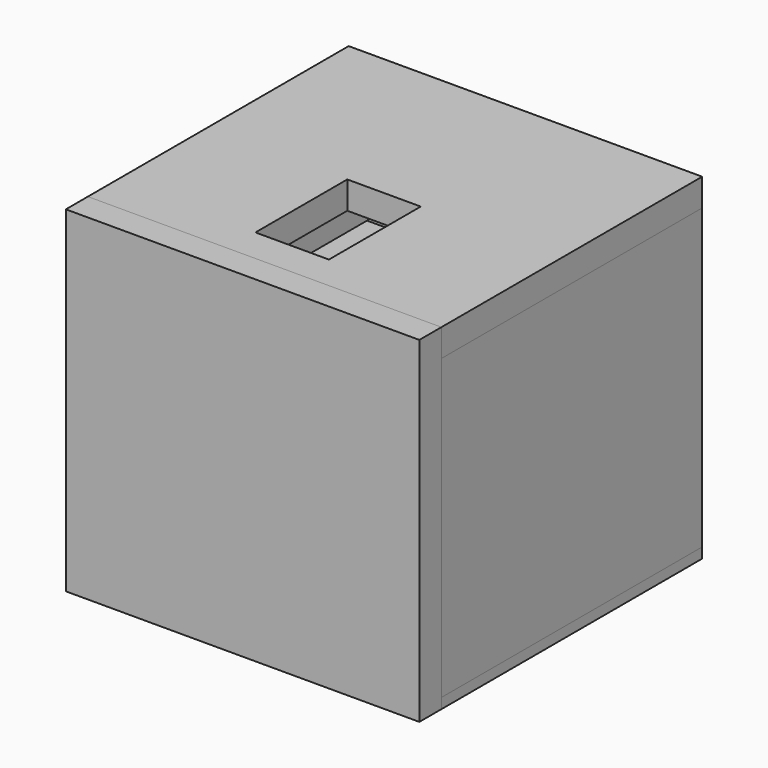
from build123d import *

# Parameters (mm, degrees)
F0_W      = 154
F0_H      = 146.5
F1_DEPTH  = 12
F2_W      = 142
F2_H      = 130
F3_DEPTH  = 12
F5_W      = 154
F5_H      = 142
F5_W_2    = 32
F5_H_2    = 50
F6_DEPTH  = 12
F7_W      = 154
F7_H      = 142
F8_DEPTH  = 4.5
F9_W      = 130
F9_H      = 130
F10_DEPTH = 4.5
F11_W     = 3
F11_H     = 3
F12_DEPTH = 142
F14_W     = 136
F14_H     = 137
F15_DEPTH = 3


# Not quite as in the source:
# - a feature names something its author has since deleted; it is built from what else it names


with BuildPart() as f1:
    # F0 (on Front) → F1 (new body)
    with BuildSketch(Plane.XZ):
        with Locations((0, 3.75)):
            Rectangle(F0_W, F0_H)
    extrude(amount=F1_DEPTH)


with BuildPart() as f3:
    # F2 (on face) → F3 (new body)
    with BuildSketch(Plane.YZ.offset(77)):
        with Locations((71, 0)):
            Rectangle(F2_W, F2_H)
    extrude(amount=-F3_DEPTH)

    # F11 (on face) → F12 (cut)
    with BuildSketch(Plane(origin=(0, 142, 0), x_dir=(-1, 0, 0), z_dir=(0, 1, 0))):
        with Locations((-66.5, 14.5)):
            Rectangle(F11_W, F11_H)
        with Locations((-66.5, -28.5)):
            Rectangle(F11_W, F11_H)
    extrude(amount=-F12_DEPTH, mode=Mode.SUBTRACT)


with BuildPart() as f4_1:
    # F4: instance of F1
    add(f1.part.mirror(Plane.YZ))


with BuildPart() as f6:
    # F5 (on face) → F6 (new body)
    with BuildSketch(Plane.XY.offset(77)):
        with Locations((0, 71)):
            Rectangle(F5_W, F5_H)
        with Locations((0, 40)):
            Rectangle(F5_W_2, F5_H_2, mode=Mode.SUBTRACT)
    extrude(amount=-F6_DEPTH)


with BuildPart() as f8:
    # F7 (on face) → F8 (new body)
    with BuildSketch(Plane(origin=(0, 0, -69.5), x_dir=(1, 0, 0), z_dir=(0, 0, -1))):
        with Locations((0, -71)):
            Rectangle(F7_W, F7_H)
    extrude(amount=-F8_DEPTH)


with BuildPart() as f10:
    # F9 (on face) → F10 (new body)
    with BuildSketch(Plane(origin=(0, 142, 0), x_dir=(-1, 0, 0), z_dir=(0, 1, 0))):
        Rectangle(F9_W, F9_H)
    extrude(amount=-F10_DEPTH)


with BuildPart() as f13_1:
    # F13: instance of F3
    add(f3.part.mirror(Plane.YZ))


with BuildPart() as f15:
    # F14 (on face) → F15 (new body)
    with BuildSketch(Plane.XY.offset(13)):
        with Locations((0, 68.5)):
            Rectangle(F14_W, F14_H)
    extrude(amount=F15_DEPTH)


with BuildPart() as f16_1:
    # F16: copy of F15
    add(f15.part.moved(Location((0, 0, -43))))


solid = Compound([f1.part, f3.part, f4_1.part, f6.part, f8.part, f10.part, f13_1.part, f15.part, f16_1.part])
